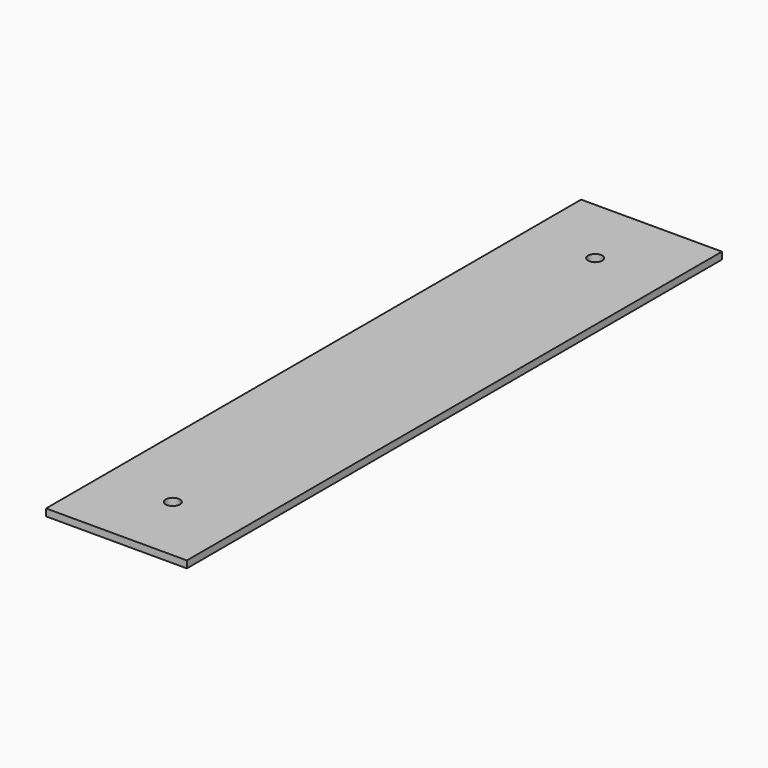
from build123d import *

# Parameters (mm, degrees)
F0_W     = 31.75
F0_H     = 31.75
F1_DEPTH = 3.175
F2_DEPTH = 3.175
F3_D     = 6.35
F3_2_D   = 6.35


# Not quite as in the source:
# - a feature names something its author has since deleted; it is built from what else it names


with BuildPart() as f1:
    # F0 (on Top) → F1 (new body)
    with BuildSketch(Plane.XY):
        Polygon((31.75, -119.0625), (31.75, 150.8125), (0, 150.8125), (0, 119.0625), (0, -119.0625), align=None)
        Polygon((0, 119.0625), (0, 150.8125), (-31.75, 150.8125), (-31.75, -119.0625), (0, -119.0625), align=None)
        with Locations((15.875, -134.9375)):
            Rectangle(F0_W, F0_H)
        with Locations((-15.875, -134.9375)):
            Rectangle(F0_W, F0_H)
    extrude(amount=F1_DEPTH)

    # F3 (through all)
    with Locations(Plane(origin=(0, 0, 0), x_dir=(1, 0, 0), z_dir=(0, 0, -1))):
        with Locations((0, 119.0625), (0, -119.0625)):
            Hole(F3_D / 2)


with BuildPart() as f2:
    # F0 (on Top) → F2 (new body)
    with BuildSketch(Plane.XY):
        Polygon((31.75, -119.0625), (31.75, 150.8125), (0, 150.8125), (0, 119.0625), (0, -119.0625), align=None)
        Polygon((0, 119.0625), (0, 150.8125), (-31.75, 150.8125), (-31.75, -119.0625), (0, -119.0625), align=None)
        with Locations((15.875, -134.9375)):
            Rectangle(F0_W, F0_H)
        with Locations((-15.875, -134.9375)):
            Rectangle(F0_W, F0_H)
    extrude(amount=F2_DEPTH)

    # F3#2 (through all)
    with Locations(Plane(origin=(0, 0, 0), x_dir=(1, 0, 0), z_dir=(0, 0, -1))):
        with Locations((0, 119.0625), (0, -119.0625)):
            Hole(F3_2_D / 2)


solid = Compound([f1.part, f2.part])
